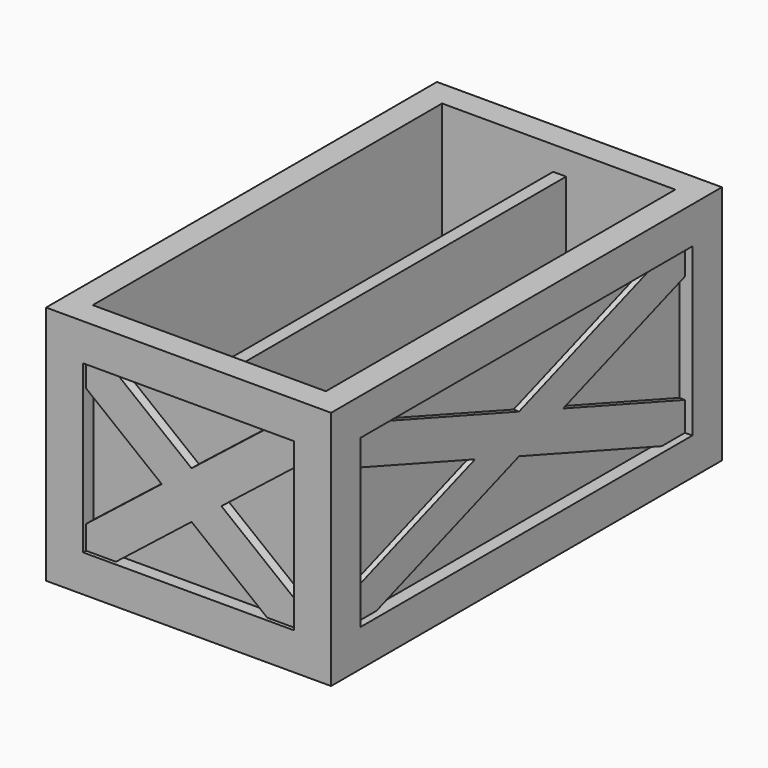
from build123d import *

# Parameters (mm, degrees)
F0_W      = 140
F0_H      = 130
F1_DEPTH  = 250
F2_W      = 126
F2_H      = 236
F3_DEPTH  = 123
F4_W      = 250
F4_H      = 130
F4_W_2    = 224
F4_H_2    = 90
F4_W_3    = 7
F5_DEPTH  = 7
F7_W      = 140
F7_H      = 130
F7_W_2    = 114
F7_H_2    = 90
F8_DEPTH  = 7
F9_W      = 140
F9_H      = 130
F9_W_2    = 114
F9_H_2    = 90
F10_DEPTH = 7
F12_DEPTH = 3
F14_DEPTH = 3
F15_W     = 7
F15_H     = 110
F16_DEPTH = 236
F18_DEPTH = 5


# Not quite as in the source:
# - a pattern or mirror of a feature is missing from the dataset's text; its kind, count and spacing are read off the source's solid


with BuildPart() as f1:
    # F0 (on Front) → F1 (new body)
    with BuildSketch(Plane.XZ):
        with Locations((70, 65)):
            Rectangle(F0_W, F0_H)
    extrude(amount=F1_DEPTH)

    # F2 (on face) → F3 (cut)
    with BuildSketch(Plane.XY.offset(130)):
        with Locations((70, -125)):
            Rectangle(F2_W, F2_H)
    extrude(amount=-F3_DEPTH, mode=Mode.SUBTRACT)

    # F4 (on face) → F5 (join)
    with BuildSketch(Plane.YZ.offset(140)):
        with Locations((-125, 65)):
            Rectangle(F4_W, F4_H)
        with Locations((-125, 65)):
            Rectangle(F4_W_2, F4_H_2, mode=Mode.SUBTRACT)
        with Locations((-253.5, 65)):
            Rectangle(F4_W_3, F4_H)
        with Locations((3.5, 65)):
            Rectangle(F4_W_3, F4_H)
    f5 = extrude(amount=F5_DEPTH)

    # F5_copies: F5 across plane
    add(f5.mirror(Plane(origin=(70, 0, 0), x_dir=(0, 0, -1), z_dir=(-1, 0, 0))))

    # F7 (on face) → F8 (join)
    with BuildSketch(Plane.XZ.offset(250)):
        with Locations((70, 65)):
            Rectangle(F7_W, F7_H)
        with Locations((70, 65)):
            Rectangle(F7_W_2, F7_H_2, mode=Mode.SUBTRACT)
    extrude(amount=F8_DEPTH)

    # F9 (on face) → F10 (join)
    with BuildSketch(Plane(origin=(0, 0, 0), x_dir=(-1, 0, 0), z_dir=(0, 1, 0))):
        with Locations((-70, 65)):
            Rectangle(F9_W, F9_H)
        with Locations((-70, 65)):
            Rectangle(F9_W_2, F9_H_2, mode=Mode.SUBTRACT)
    extrude(amount=F10_DEPTH)

    # F11 (on face) → F12 (join)
    with BuildSketch(Plane.YZ.offset(140)):
        Polygon((-13, 35.6504185324), (-221.3495814676, 110), (-237, 110), (-237, 94.3495814676), (-28.6504185324, 20), (-13, 20), align=None)
    f12 = extrude(amount=F12_DEPTH)

    # F12_copies: F12 across plane
    add(f12.mirror(Plane(origin=(70, 0, 0), x_dir=(0, 0, -1), z_dir=(-1, 0, 0))))

    # F13 (on face) → F14 (join)
    with BuildSketch(Plane.YZ.offset(140)):
        Polygon((-13, 110), (-28.6504185324, 110), (-237, 35.6504185324), (-237, 20), (-221.3495814676, 20), (-13, 94.3495814676), align=None)
    f14 = extrude(amount=F14_DEPTH)

    # F14_copies: F14 across plane
    add(f14.mirror(Plane(origin=(70, 0, 0), x_dir=(0, 0, -1), z_dir=(-1, 0, 0))))

    # F15 (on face) → F16 (join, through all)
    with BuildSketch(Plane.XZ.offset(7)):
        with Locations((70.5, 62)):
            Rectangle(F15_W, F15_H)
    extrude(amount=F16_DEPTH)

    # F17 (on face) → F18 (join)
    with BuildSketch(Plane.XZ.offset(250)):
        Polygon((70, 77.7407562494), (29.1382912492, 110), (13, 110), (13, 97.2592437506), (53.8617087508, 65), (13, 32.7407562494), (13, 20), (29.1382912492, 20), (70, 52.2592437506), (110.8617087508, 20), (127, 20), (127, 32.7407562494), (86.1382912492, 65), (127, 97.2592437506), (127, 110), (110.8617087508, 110), align=None)
    f18 = extrude(amount=F18_DEPTH)

    # F18_copies: F18 across plane
    add(f18.mirror(Plane.ZX.offset(-125)))


solid = f1.part
